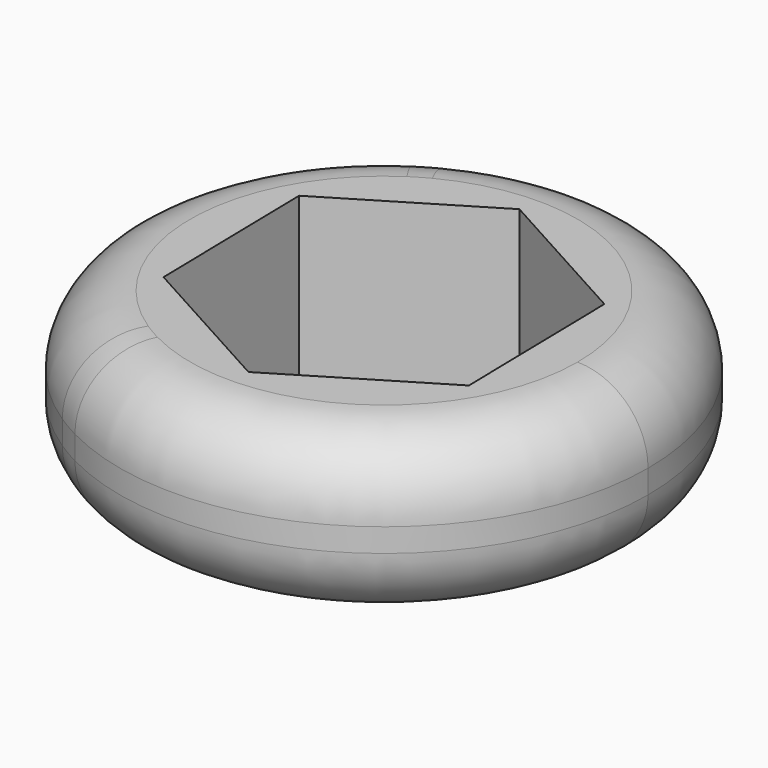
from build123d import *

# Parameters (mm, degrees)
F1_DEPTH = 7
F2_R     = 3


# Not quite as in the source:
# - a feature names something its author has since deleted; it is built from what else it names


with BuildPart() as f1:
    # F0 (on Top) → F1 (new body)
    with BuildSketch(Plane.XY):
        with BuildLine():
            ThreePointArc((19.8306639352, -9.9816080654), (30.8415453201, -9.6036911235), (36.2407533076, 0))
            ThreePointArc((36.2407533076, 0), (30.8415453201, 9.6036911235), (19.8306639352, 9.9816080654))
            ThreePointArc((19.8306639352, 9.9816080654), (19.3470475071, 9.6503015364), (18.8215508103, 9.3904898984))
            ThreePointArc((18.8215508103, 9.3904898984), (13.7592466924, 0), (18.8215508103, -9.3904898984))
            ThreePointArc((18.8215508103, -9.3904898984), (19.3470475071, -9.6503015364), (19.8306639352, -9.9816080654))
        make_face()
        Polygon((31.3263880982, 3.8197050887), (31.4711556909, -3.5689602629), (25.1447675927, -7.3886653516), (18.6736119018, -3.8197050887), (18.5288443091, 3.5689602629), (24.8552324073, 7.3886653516), align=None, mode=Mode.SUBTRACT)
        with BuildLine():
            ThreePointArc((18.8215508103, -9.3904898984), (19.3184145947, -9.6991815224), (19.8306639352, -9.9816080654))
            ThreePointArc((19.8306639352, -9.9816080654), (19.3470475071, -9.6503015364), (18.8215508103, -9.3904898984))
        make_face()
        with BuildLine():
            ThreePointArc((18.8215508103, 9.3904898984), (19.3470475071, 9.6503015364), (19.8306639352, 9.9816080654))
            ThreePointArc((19.8306639352, 9.9816080654), (19.3184145947, 9.6991815224), (18.8215508103, 9.3904898984))
        make_face()
    extrude(amount=F1_DEPTH)

    # F2
    f2_edges = [f1.edges().sort_by_distance(p)[0] for p in [
        (31.178449, -9.39049, 7),
        (31.178449, -9.39049, 0),
    ]]
    fillet(f2_edges, radius=F2_R)


solid = f1.part
